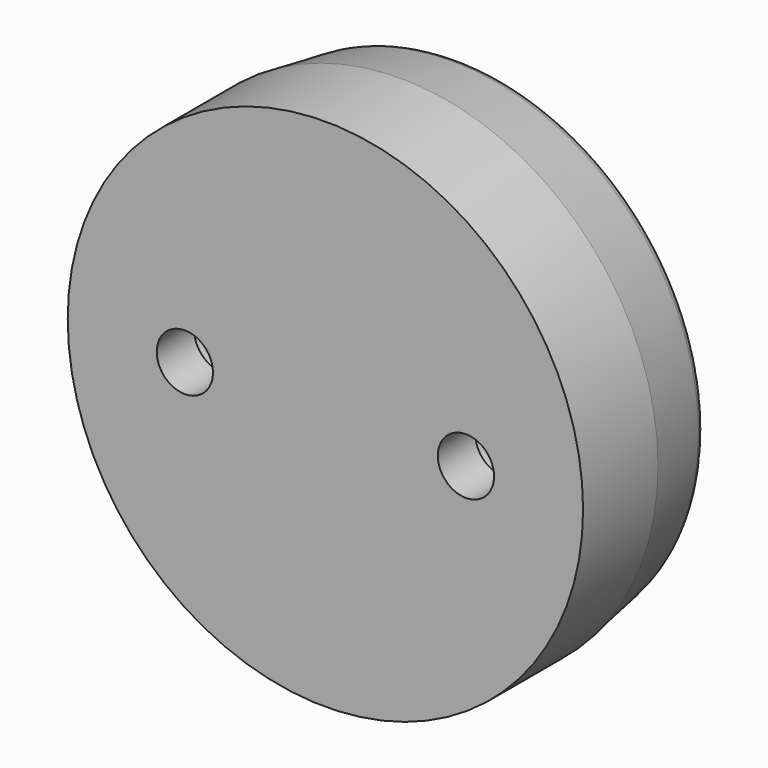
from build123d import *

# Parameters (mm, degrees)
F2_R      = 0.5
F5_DEPTH  = 5
F6_R      = 0.5
F7_R      = 2
F8_DEPTH  = 7
F9_R      = 1.2
F10_DEPTH = 25


with BuildPart() as f1:
    # F0 (on Top) → F1 (revolve)
    with BuildSketch(Plane.XY):
        with BuildLine():
            Line((0, 9), (0, 0))
            Line((0, 0), (11, 0))
            Line((11, 0), (11, 4))
            Line((11, 4), (10.5, 7))
            ThreePointArc((10.5, 7), (10.0017468007, 7.1915925315), (9.5, 7.3738398822))
            Line((9.5, 7.3738398822), (9.5, 6.5449972332))
            Line((9.5, 6.5449972332), (9, 6.5449972332))
            Line((9, 6.5449972332), (9, 7.5449972332))
            ThreePointArc((9, 7.5449972332), (4.5584271698, 8.6339031037), (0, 9))
        make_face()
    revolve(axis=Axis((0, 4.5, 0), (0, -1, 0)))

    # F2
    f2_edges = [f1.edges().sort_by_distance(p)[0] for p in [
        (-10.5, 7, 0),
    ]]
    fillet(f2_edges, radius=F2_R)

    # F4 (on offset) → F5 (cut)
    with BuildSketch(Plane.XZ.offset(-9)):
        with BuildLine():
            ThreePointArc((-4.905379299, -6.3195928613), (5.6568542495, -5.6568542495), (6.3195928613, 4.905379299))
            Line((6.3195928613, 4.905379299), (-4.905379299, -6.3195928613))
        make_face()
        with BuildLine():
            Line((-6.3195928613, -4.905379299), (4.905379299, 6.3195928613))
            ThreePointArc((4.905379299, 6.3195928613), (-5.6568542495, 5.6568542495), (-6.3195928613, -4.905379299))
        make_face()
    extrude(amount=F5_DEPTH, mode=Mode.SUBTRACT)

    # F6
    f6_edges = [f1.edges().sort_by_distance(p)[0] for p in [
        (6.319593, 5.928385, 4.905379),
        (-4.905379, 5.928385, -6.319593),
        (-6.319593, 5.928385, -4.905379),
        (4.905379, 5.928385, 6.319593),
    ]]
    fillet(f6_edges, radius=F6_R)

    # F7 (on offset) → F8 (cut)
    with BuildSketch(Plane.XZ.offset(-9)):
        with Locations((6, 0)):
            Circle(F7_R)
        with Locations((-6, 0)):
            Circle(F7_R)
    extrude(amount=F8_DEPTH, mode=Mode.SUBTRACT)

    # F9 (on face) → F10 (cut)
    with BuildSketch(Plane(origin=(0, 2, 0), x_dir=(-1, 0, 0), z_dir=(0, 1, 0))):
        with Locations((-6, 0)):
            Circle(F9_R)
        with Locations((6, 0)):
            Circle(F9_R)
    extrude(amount=-F10_DEPTH, mode=Mode.SUBTRACT)


solid = f1.part
